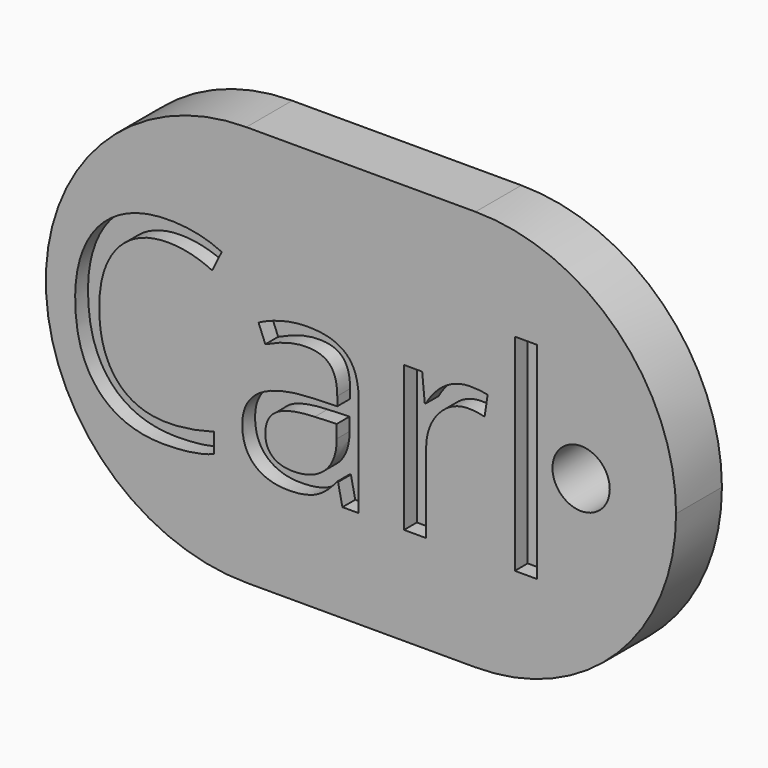
from build123d import *

# Parameters (mm, degrees)
F1_DEPTH     = 6.35
F2_R         = 3.175
F3_DEPTH     = 25.4
F4_TEXT_SIZE = 30.0760122223
F5_DEPTH     = 1.778


# Not quite as in the source:
# - Text() gives the source's letters only with a copy of the font that has no kerning and outlines rounded to 1/6400 em; it was checked with that copy


with BuildPart() as f1:
    # F0 (on Front) → F1 (new body)
    with BuildSketch(Plane.XZ):
        with BuildLine():
            ThreePointArc((22.225, 0), (19.700356913, 10.2881758587), (12.7, 18.2389864028))
            ThreePointArc((12.7, 18.2389864028), (3.175, 0), (12.7, -18.2389864028))
            ThreePointArc((12.7, -18.2389864028), (19.700356913, -10.2881758587), (22.225, 0))
        make_face()
        with BuildLine():
            Line((25.4, 22.225), (0, 22.225))
            ThreePointArc((0, 22.225), (6.6554170492, 21.2050948807), (12.7, 18.2389864028))
            ThreePointArc((12.7, 18.2389864028), (18.7445829508, 21.2050948807), (25.4, 22.225))
        make_face()
        with BuildLine():
            ThreePointArc((12.7, -18.2389864028), (6.6554170492, -21.2050948807), (0, -22.225))
            Line((0, -22.225), (25.4, -22.225))
            ThreePointArc((25.4, -22.225), (18.7445829508, -21.2050948807), (12.7, -18.2389864028))
        make_face()
        with BuildLine():
            ThreePointArc((12.7, 18.2389864028), (6.6554170492, 21.2050948807), (0, 22.225))
            ThreePointArc((0, 22.225), (-22.225, 0), (0, -22.225))
            ThreePointArc((0, -22.225), (6.6554170492, -21.2050948807), (12.7, -18.2389864028))
            ThreePointArc((12.7, -18.2389864028), (3.175, 0), (12.7, 18.2389864028))
        make_face()
        with BuildLine():
            ThreePointArc((25.4, 22.225), (18.7445829508, 21.2050948807), (12.7, 18.2389864028))
            ThreePointArc((12.7, 18.2389864028), (19.700356913, 10.2881758587), (22.225, 0))
            ThreePointArc((22.225, 0), (19.700356913, -10.2881758587), (12.7, -18.2389864028))
            ThreePointArc((12.7, -18.2389864028), (18.7445829508, -21.2050948807), (25.4, -22.225))
            ThreePointArc((25.4, -22.225), (41.1154482119, -15.7154482119), (47.625, 0))
            ThreePointArc((47.625, 0), (41.1154482119, 15.7154482119), (25.4, 22.225))
        make_face()
    extrude(amount=F1_DEPTH)

    # F2 (on face) → F3 (cut)
    with BuildSketch(Plane.XZ.offset(6.35)):
        with Locations((37.099210749, 0)):
            Circle(F2_R)
    extrude(amount=-F3_DEPTH, mode=Mode.SUBTRACT)

    # F4 (on face) → F5 (cut)
    with BuildSketch(Plane.XZ.offset(6.35)):
        with Locations((-20.8110380918, -11.3898236305)):
            Text('Carl', F4_TEXT_SIZE, font='Open Sans', text_align=(TextAlign.LEFT, TextAlign.BOTTOM))
    extrude(amount=-F5_DEPTH, mode=Mode.SUBTRACT)


solid = f1.part
